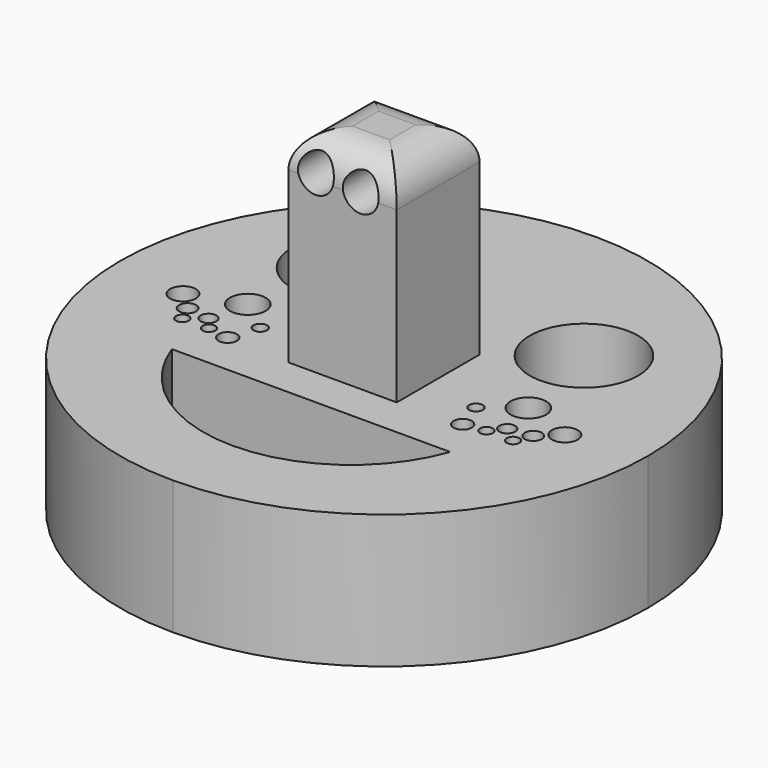
from build123d import *

# Parameters (mm, degrees)
F0_R        = 0.9128432721
F0_R_2      = 1.2216898107
F0_R_3      = 1.8377143243
F0_R_4      = 1.1282865395
F0_R_5      = 1.3035270966
F0_R_6      = 0.9702753
F0_R_7      = 2.5484542397
F0_R_8      = 7.7130109431
F1_DEPTH    = 19.05
F2_DEPTH    = 48.26
F4_D        = 5.08
F4_DEPTH    = 12.7
F4_TIP      = 1.5261859723
F5_T1_DEPTH = 40.8239460826
F5_T3_DEPTH = 40.1487670183


# Not quite as in the source:
# - a fillet or chamfer that OpenCascade refuses, or shapes differently, is made with other operations: its cross-section is extruded or revolved along the edge and cut away or added


with BuildPart() as f1:
    # F0 (on Top) → F1 (new body)
    with BuildSketch(Plane.XY):
        with BuildLine():
            Line((-46.1318939924, 34.7651951015), (-46.1318939924, 64.978521944))
            ThreePointArc((-46.1318939924, 64.978521944), (-83.7196043441, 27.3908115923), (-46.1318939924, -10.1968987593))
            Line((-46.1318939924, -10.1968987593), (-46.1318939924, 0.4695183748))
            ThreePointArc((-46.1318939924, 0.4695183748), (-58.2504121537, 4.3055568595), (-65.9541934729, 14.4162159413))
            Line((-65.9541934729, 14.4162159413), (-46.1318939924, 14.4162159413))
            Line((-46.1318939924, 14.4162159413), (-46.1318939924, 20.0164280832))
            Line((-46.1318939924, 20.0164280832), (-53.8438670337, 20.0164280832))
            Line((-53.8438670337, 20.0164280832), (-53.8438670337, 34.7651951015))
            Line((-53.8438670337, 34.7651951015), (-46.1318939924, 34.7651951015))
        make_face()
        with Locations((-69.6755722165, 20.9292713553)):
            Circle(F0_R, mode=Mode.SUBTRACT)
        with Locations((-65.8872798085, 20.9292713553)):
            Circle(F0_R, mode=Mode.SUBTRACT)
        with Locations((-70.7362964749, 23.2022479177)):
            Circle(F0_R_2, mode=Mode.SUBTRACT)
        with Locations((-73.3180493116, 25.5887825042)):
            Circle(F0_R_3, mode=Mode.SUBTRACT)
        with Locations((-67.4026012421, 22.7476526052)):
            Circle(F0_R_4, mode=Mode.SUBTRACT)
        with Locations((-62.856644392, 20.4746760428)):
            Circle(F0_R_5, mode=Mode.SUBTRACT)
        with Locations((-61.4928565919, 24.5660338551)):
            Circle(F0_R_6, mode=Mode.SUBTRACT)
        with Locations((-66.1099404097, 28.1116217375)):
            Circle(F0_R_7, mode=Mode.SUBTRACT)
        with Locations((-63.0709454417, 41.807025671)):
            Circle(F0_R_8, mode=Mode.SUBTRACT)
        with BuildLine():
            ThreePointArc((-46.1318939924, -10.1968987593), (-19.5533691135, 0.8122867134), (-8.5441836408, 27.3908115923))
            ThreePointArc((-8.5441836408, 27.3908115923), (-19.5533691135, 53.9693364713), (-46.1318939924, 64.978521944))
            Line((-46.1318939924, 64.978521944), (-46.1318939924, 34.7651951015))
            Line((-46.1318939924, 34.7651951015), (-38.4199209511, 34.7651951015))
            Line((-38.4199209511, 34.7651951015), (-38.4199209511, 20.0164280832))
            Line((-38.4199209511, 20.0164280832), (-46.1318939924, 20.0164280832))
            Line((-46.1318939924, 20.0164280832), (-46.1318939924, 14.4162159413))
            Line((-46.1318939924, 14.4162159413), (-26.309594512, 14.4162159413))
            ThreePointArc((-26.309594512, 14.4162159413), (-34.0133758311, 4.3055568595), (-46.1318939924, 0.4695183748))
            Line((-46.1318939924, 0.4695183748), (-46.1318939924, -10.1968987593))
        make_face()
        with Locations((-29.4071435928, 20.4746760428)):
            Circle(F0_R_5, mode=Mode.SUBTRACT)
        with Locations((-30.7709313929, 24.5660338551)):
            Circle(F0_R_6, mode=Mode.SUBTRACT)
        with Locations((-26.3765081763, 20.9292713553)):
            Circle(F0_R, mode=Mode.SUBTRACT)
        with Locations((-22.5882157683, 20.9292713553)):
            Circle(F0_R, mode=Mode.SUBTRACT)
        with Locations((-24.8611867428, 22.7476526052)):
            Circle(F0_R_4, mode=Mode.SUBTRACT)
        with Locations((-21.5274915099, 23.2022479177)):
            Circle(F0_R_2, mode=Mode.SUBTRACT)
        with Locations((-18.9457386732, 25.5887825042)):
            Circle(F0_R_3, mode=Mode.SUBTRACT)
        with Locations((-29.1928425431, 41.807025671)):
            Circle(F0_R_8, mode=Mode.SUBTRACT)
        with Locations((-26.1538475752, 28.1116217375)):
            Circle(F0_R_7, mode=Mode.SUBTRACT)
    extrude(amount=F1_DEPTH)

    # F0 (on Top) → F2 (join)
    with BuildSketch(Plane.XY):
        Polygon((-38.4199209511, 34.7651951015), (-46.1318939924, 34.7651951015), (-46.1318939924, 27.3908115923), (-46.1318939924, 20.0164280832), (-38.4199209511, 20.0164280832), align=None)
        Polygon((-46.1318939924, 27.3908115923), (-46.1318939924, 34.7651951015), (-53.8438670337, 34.7651951015), (-53.8438670337, 20.0164280832), (-46.1318939924, 20.0164280832), align=None)
    extrude(amount=F2_DEPTH)

    # F4
    with Locations(Plane.XZ.offset(-20.0164280832)):
        with Locations((-49.9697290361, 43.8477247953), (-43.5725338757, 43.5774177313)):
            Hole(F4_D / 2, depth=F4_DEPTH)
            with Locations((0, 0, -(F4_DEPTH + F4_TIP / 2))):  # 118° drill point
                Cone(0, F4_D / 2, F4_TIP, mode=Mode.SUBTRACT)

    # F5: fillet of radius 5.08 on 4 edges, made by hand

    # F5_s2 → F5_t1 (cut)
    with BuildSketch(Plane.YZ.offset(-66.5438670337)):
        with BuildLine():
            ThreePointArc((34.7651951015, 43.18), (33.2772975499, 46.7721024484), (29.6851951015, 48.26))
            Line((29.6851951015, 48.26), (34.7651951015, 48.26))
            Line((34.7651951015, 48.26), (34.7651951015, 43.18))
        make_face()
        with BuildLine():
            ThreePointArc((20.0164280832, 43.18), (21.5043256348, 46.7721024484), (25.0964280832, 48.26))
            Line((25.0964280832, 48.26), (20.0164280832, 48.26))
            Line((20.0164280832, 48.26), (20.0164280832, 43.18))
        make_face()
    extrude(amount=F5_T1_DEPTH, mode=Mode.SUBTRACT)

    # F5_s4 → F5_t3 (cut)
    with BuildSketch(Plane.XZ.offset(-47.4651951015)):
        with BuildLine():
            ThreePointArc((-53.8438670337, 43.18), (-52.3559694821, 46.7721024484), (-48.7638670337, 48.26))
            Line((-48.7638670337, 48.26), (-53.8438670337, 48.26))
            Line((-53.8438670337, 48.26), (-53.8438670337, 43.18))
        make_face()
        with BuildLine():
            ThreePointArc((-38.4199209511, 43.18), (-39.9078185027, 46.7721024484), (-43.4999209511, 48.26))
            Line((-43.4999209511, 48.26), (-38.4199209511, 48.26))
            Line((-38.4199209511, 48.26), (-38.4199209511, 43.18))
        make_face()
    extrude(amount=F5_T3_DEPTH, mode=Mode.SUBTRACT)


solid = f1.part
